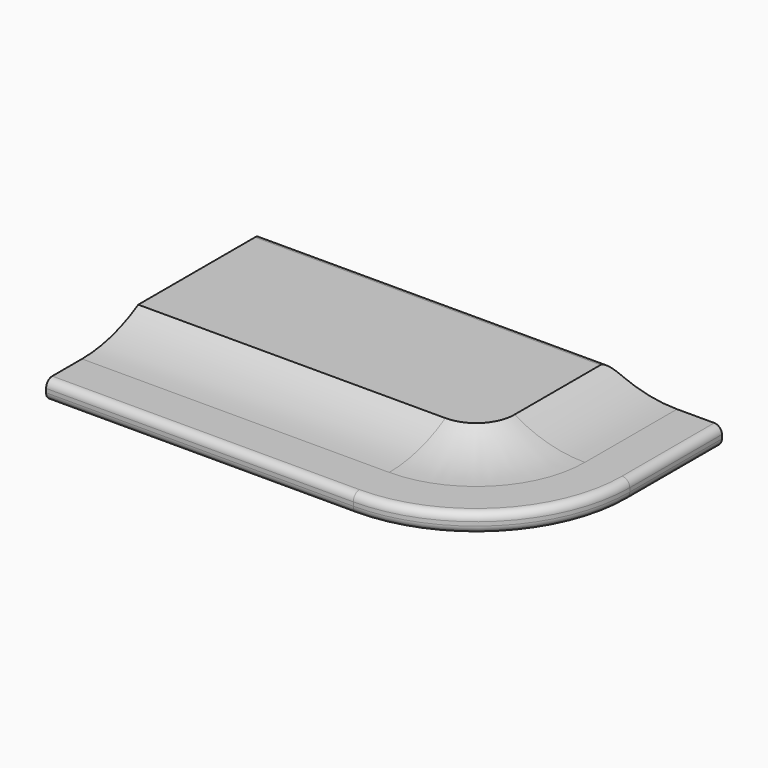
from build123d import *

# Parameters (mm, degrees)
F1_DEPTH = 4.7625
F8_DEPTH = 25.4
F9_R     = 1.27


with BuildPart() as f1:
    # F0 (on Top) → F1 (new body, symmetric)
    with BuildSketch(Plane.XY):
        with BuildLine():
            Line((0, 44.45), (0, 0))
            Line((0, 0), (50.8, 0))
            ThreePointArc((50.8, 0), (68.7605122421, 7.4394877579), (76.2, 25.4))
            Line((76.2, 25.4), (76.2, 44.45))
            Line((76.2, 44.45), (0, 44.45))
        make_face()
    extrude(amount=F1_DEPTH, both=True)


with BuildPart() as f4:
    # F4: sweep along a path in F3
    with BuildLine(Plane.XY.offset(4.7625)) as f4_path:
        Line((0, 0), (50.8, 0))
        ThreePointArc((50.8, 0), (68.7605122421, 7.4394877579), (76.2, 25.4))
        Line((76.2, 25.4), (76.2, 44.45))
    # F2 (on face) → F4 (sweep)
    with BuildSketch(Plane(origin=(0, 0, 0), x_dir=(0, -1, 0), z_dir=(-1, 0, 0))):
        with BuildLine():
            Line((0, 4.7625), (-19.05, 4.7625))
            ThreePointArc((-19.05, 4.7625), (-13.4517306294, 2.3955307002), (-7.4275916867, 1.5875))
            Line((-7.4275916867, 1.5875), (0, 1.5875))
            Line((0, 1.5875), (0, 4.7625))
        make_face()
    sweep(path=f4_path.line)


with BuildPart() as f5_1:
    # F5: instance of F4
    add(f4.part.mirror(Plane.XY))


with BuildPart() as f1_1:
    add(f1.part)

    # F6: cut F4, F5_1
    add(f4.part, mode=Mode.SUBTRACT)
    add(f5_1.part, mode=Mode.SUBTRACT)

    # F7 (on face) → F8 (cut)
    with BuildSketch(Plane(origin=(0, 0, 0), x_dir=(0, -1, 0), z_dir=(-1, 0, 0))):
        with BuildLine():
            Line((-38.1, -3.175), (-25.4, -3.175))
            ThreePointArc((-25.4, -3.175), (-23.1549359697, -2.2450640303), (-22.225, 0))
            ThreePointArc((-22.225, 0), (-23.1549359697, 2.2450640303), (-25.4, 3.175))
            Line((-25.4, 3.175), (-38.1, 3.175))
            ThreePointArc((-38.1, 3.175), (-40.3450640303, 2.2450640303), (-41.275, 0))
            ThreePointArc((-41.275, 0), (-40.3450640303, -2.2450640303), (-38.1, -3.175))
        make_face()
    extrude(amount=-F8_DEPTH, mode=Mode.SUBTRACT)

    # F9
    f9_edges = [f1_1.edges().sort_by_distance(p)[0] for p in [
        (28.575, 44.45, 4.7625),
        (28.575, 44.45, -4.7625),
        (25.4, 0, 1.5875),
        (68.760512, 7.439488, 1.5875),
        (76.2, 34.925, 1.5875),
        (25.4, 0, -1.5875),
        (68.760512, 7.439488, -1.5875),
        (76.2, 34.925, -1.5875),
    ]]
    fillet(f9_edges, radius=F9_R)


solid = f1_1.part
